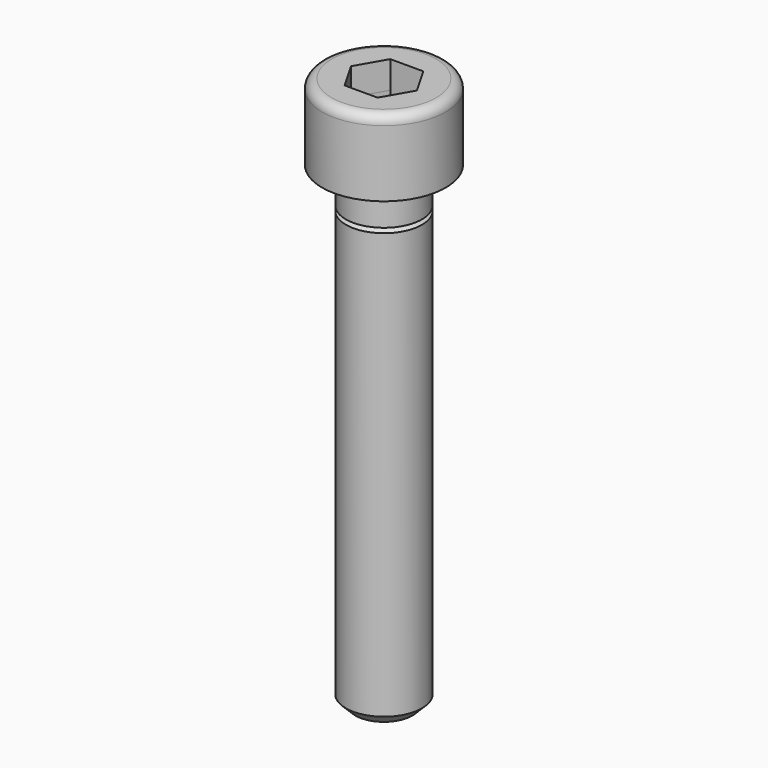
from build123d import *

# Parameters (mm, degrees)
F2_R     = 1
F3_SIZE  = 1
F5_DEPTH = 2.88


# Not quite as in the source:
# - a fillet or chamfer that OpenCascade refuses, or shapes differently, is made with other operations: its cross-section is extruded or revolved along the edge and cut away or added


with BuildPart() as f1:
    # F0 (on Front) → F1 (revolve)
    with BuildSketch(Plane.XZ):
        Polygon((-4, 0), (0, 0), (0, 51.056624327), (-2.5, 52.5), (-2.5, 58), (-6.5, 58), (-6.5, 50), (-4, 50), (-4, 46.25), (-3.5, 46), (-4, 45.75), align=None)
    revolve(axis=Axis((0, 0, 18.332445994), (0, 0, 1)))

    # F2
    f2_edges = [f1.edges().sort_by_distance(p)[0] for p in [
        (6.5, 0, 58),
    ]]
    fillet(f2_edges, radius=F2_R)

    # F3
    f3_edges = [f1.edges().sort_by_distance(p)[0] for p in [
        (4, 0, 0),
    ]]
    chamfer(f3_edges, length=F3_SIZE)

    # F4 (on face) → F5 (cut)
    with BuildSketch(Plane.XY.offset(58)):
        Polygon((-1.7320508076, -3), (1.7320508076, -3), (3.4641016151, 0), (1.7320508076, 3), (-1.7320508076, 3), (-3.4641016151, 0), align=None)
    extrude(amount=-F5_DEPTH, mode=Mode.SUBTRACT)

    # F6: chamfer of 1.5 x 2.5980762114 on 1 edges, made by hand


with BuildPart() as f6_tool2:
    # F6_s3 → F6_t4 (revolve)
    with BuildSketch(Plane.XZ):
        Polygon((-5.0980762114, 55.12), (-2.5, 53.62), (-2.5, 55.12), align=None)
    revolve(axis=Axis((0, 0, 55.12), (0, 0, 1)))

    split(bisect_by=Plane(origin=(-2.5980762114, -1.5, 0), x_dir=(0, 0, 1), z_dir=(0.8660254038, 0.5, 0)), keep=Keep.TOP)

    split(bisect_by=Plane(origin=(-2.5980762114, 1.5, 0), x_dir=(0, 0, 1), z_dir=(0.8660254038, -0.5, 0)), keep=Keep.TOP)

    split(bisect_by=Plane.XZ.offset(-3), keep=Keep.TOP)

    split(bisect_by=Plane(origin=(2.5980762114, 1.5, 0), x_dir=(0, 0, 1), z_dir=(-0.8660254038, -0.5, 0)), keep=Keep.TOP)

    split(bisect_by=Plane(origin=(2.5980762114, -1.5, 0), x_dir=(0, 0, 1), z_dir=(-0.8660254038, 0.5, 0)), keep=Keep.TOP)

    split(bisect_by=Plane.XZ.offset(3), keep=Keep.BOTTOM)


with BuildPart() as f1_1:
    add(f1.part)

    # F6_t1: cut F6_tool2
    add(f6_tool2.part, mode=Mode.SUBTRACT)


solid = f1_1.part
